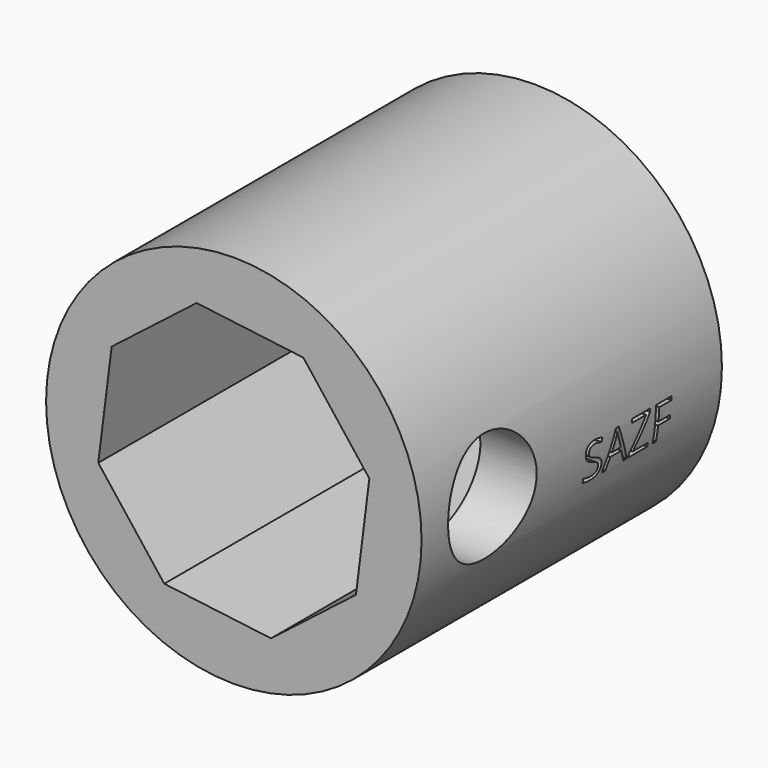
from build123d import *

# Parameters (mm, degrees)
F0_R         = 50
F1_DEPTH     = 100
F3_DEPTH     = 100.001
F4_R         = 14.7465898969
F5_DEPTH     = 69.6
F6_TEXT_SIZE = 13.0238438336
F7_DEPTH     = 76.7


# Not quite as in the source:
# - Text() gives the source's letters only with a copy of the font that has no kerning and outlines rounded to 1/6400 em; it was checked with that copy


with BuildPart() as f1:
    # F0 (on Front) → F1 (new body)
    with BuildSketch(Plane.XZ):
        Circle(F0_R)
    extrude(amount=F1_DEPTH)

    # F2 (on Front) → F3 (cut, through all)
    with BuildSketch(Plane.XZ):
        Polygon((36.0986158435, 9.8993677624), (18.5256659801, 32.5254861287), (-9.8993677624, 36.0986158435), (-32.5254861287, 18.5256659801), (-36.0986158435, -9.8993677624), (-18.5256659801, -32.5254861287), (9.8993677624, -36.0986158435), (32.5254861287, -18.5256659801), align=None)
    extrude(amount=F3_DEPTH, mode=Mode.SUBTRACT)

    # F4 (on Right) → F5 (cut)
    with BuildSketch(Plane.YZ):
        with Locations((-76.4104053378, 0)):
            Circle(F4_R)
    extrude(amount=F5_DEPTH, mode=Mode.SUBTRACT)

    # F6 (on Right) → F7 (cut)
    with BuildSketch(Plane.YZ):
        with Locations((-46.0551257727, -9.3771675602)):
            Text('SAZF', F6_TEXT_SIZE, font='Open Sans', text_align=(TextAlign.LEFT, TextAlign.BOTTOM))
    extrude(amount=F7_DEPTH, mode=Mode.SUBTRACT)


solid = f1.part
